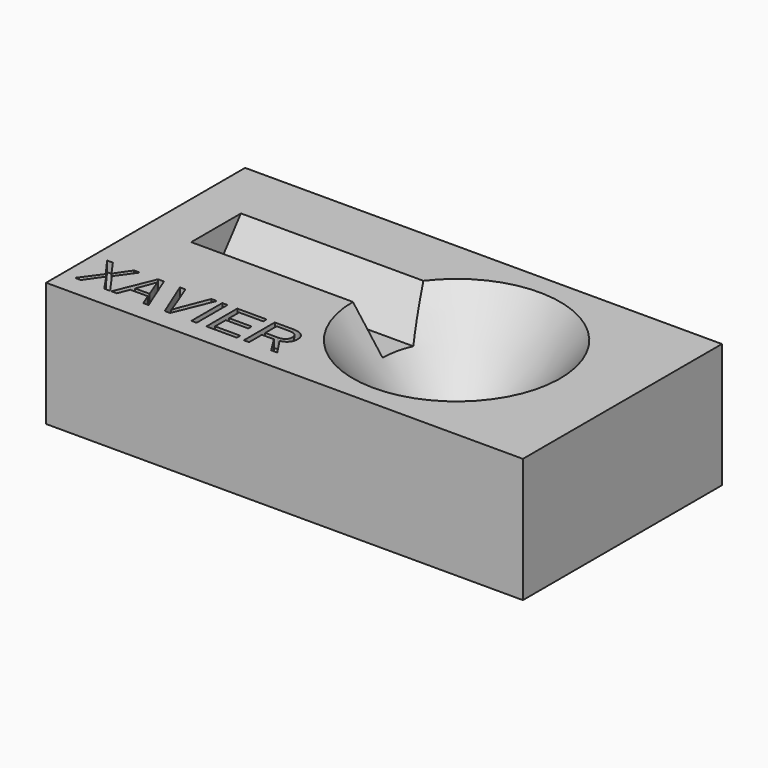
from build123d import *

# Parameters (mm, degrees)
F1_DEPTH     = 38.1
F5_DEPTH     = 76.2
F6_TEXT_SIZE = 17.2035727892
F7_DEPTH     = 3.175
F9_DEPTH     = 13.97


# Not quite as in the source:
# - Text() gives the source's letters only with a copy of the font that has no kerning and outlines rounded to 1/6400 em; it was checked with that copy


with BuildPart() as f1:
    # F0 (on Top) → F1 (new body)
    with BuildSketch(Plane.XY):
        Polygon((50.8, -38.1), (50.8, -0.3377659667), (50.8, 38.1), (-95.25, 38.1), (-95.25, -38.1), align=None)
    extrude(amount=-F1_DEPTH)

    # F2 (on Front) → F3 (revolve, cut)
    with BuildSketch(Plane.XZ):
        Polygon((0, -25.4), (0, 0), (-31.75, 0), (-12.7, -25.4), align=None)
    revolve(axis=Axis((0, 0, -12.7), (0, 0, 1)), mode=Mode.SUBTRACT)

    # F4 (on face) → F5 (cut)
    with BuildSketch(Plane(origin=(-95.25, 0, 0), x_dir=(0, -1, 0), z_dir=(-1, 0, 0))):
        Polygon((0, 0), (-19.05, 0), (-9.271, -12.1282860637), (0, -12.1282860637), align=None)
    extrude(amount=-F5_DEPTH, mode=Mode.SUBTRACT)

    # F6 (on face) → F7 (cut)
    with BuildSketch(Plane.XY):
        with Locations((-91.7905269039, -31.8217522455)):
            Text('XAVIER', F6_TEXT_SIZE, font='Arimo', text_align=(TextAlign.LEFT, TextAlign.BOTTOM))
    extrude(amount=-F7_DEPTH, mode=Mode.SUBTRACT)

    # F8 (on face) → F9 (join)
    with BuildSketch(Plane(origin=(-95.25, 0, 0), x_dir=(0, -1, 0), z_dir=(-1, 0, 0))):
        Polygon((0, 0), (-19.05, 0), (-9.271, -12.1282860637), (0, -12.1282860637), align=None)
    extrude(amount=-F9_DEPTH)


solid = f1.part
